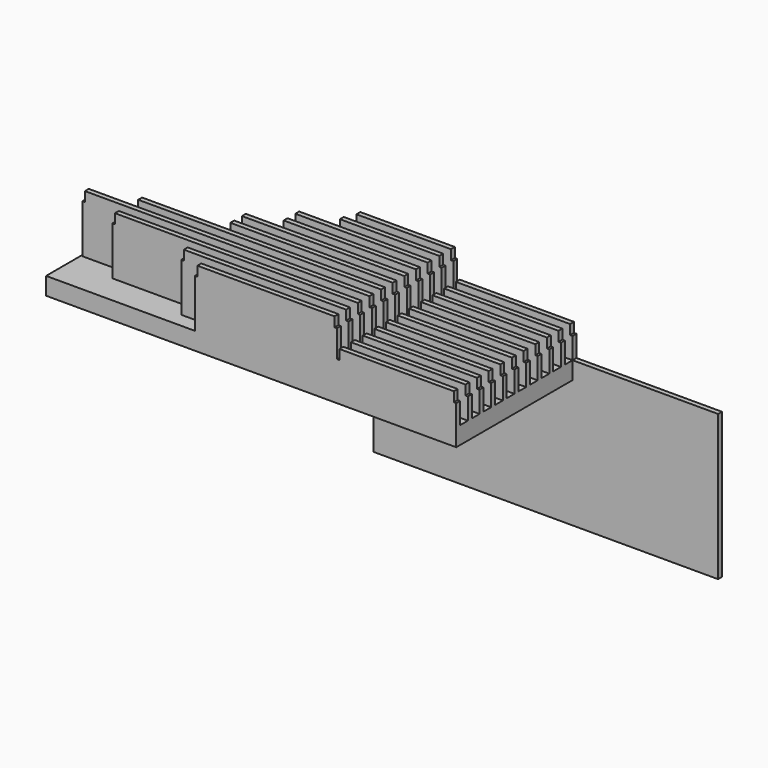
from build123d import *

# Parameters (mm, degrees)
F1_DEPTH  = 123
F2_DEPTH  = 300
F3_R      = 0.5
F4_DEPTH  = 1
F5_W      = 123
F5_H      = 28
F6_DEPTH  = 300
F7_W      = 2.5
F7_H      = 10
F8_DEPTH  = 300
F9_W      = 150
F9_H      = 150
F10_DEPTH = 5
F11_W     = 5
F11_H     = 60
F12_DEPTH = 197.5
F13_W     = 20
F13_H     = 60
F14_DEPTH = 158.5
F15_W     = 20
F15_H     = 60
F15_W_2   = 5
F16_DEPTH = 127.5
F17_W     = 5
F17_H     = 60
F18_DEPTH = 44.5
F19_W     = 5
F19_H     = 60
F20_DEPTH = 1.5
F21_W     = 5
F21_H     = 60
F22_DEPTH = 153.5
F23_W     = 5
F23_H     = 10
F24_DEPTH = 2.5
F25_W     = 5
F25_H     = 10
F26_DEPTH = 2.5
F27_W     = 5
F27_H     = 10
F28_DEPTH = 2.5
F29_W     = 5
F29_H     = 10
F30_DEPTH = 2.5
F31_W     = 5
F31_H     = 10
F32_DEPTH = 2.5
F33_W     = 5
F33_H     = 10
F34_DEPTH = 2.5
F35_W     = 5
F35_H     = 10
F36_DEPTH = 2.5
F37_W     = 5
F37_H     = 10
F38_DEPTH = 2.5
F39_W     = 5
F39_H     = 10
F40_DEPTH = 2.5
F41_W     = 5
F41_H     = 10
F42_DEPTH = 2.5
F43_W     = 5
F43_H     = 10
F44_DEPTH = 2.5
F45_W     = 217.5729006529
F45_H     = 131.9425046444
F46_DEPTH = 5


# Not quite as in the source:
# - a feature names something its author has since deleted; it is built from what else it names


with BuildPart() as f1:
    # F0 (on Right) → F1 (new body)
    with BuildSketch(Plane.YZ):
        Polygon((179.2768240368, 60), (174.2768240368, 60), (174.2768240368, -18.0574953556), (324.2768240368, -18.0574953556), (324.2768240368, -150), (329.2768240368, -150), (329.2768240368, 60), (324.2768240368, 60), (324.2768240368, 0), (314.2768240368, 0), (314.2768240368, 60), (309.2768240368, 60), (309.2768240368, 0), (299.2768240368, 0), (299.2768240368, 60), (294.2768240368, 60), (294.2768240368, 0), (284.2768240368, 0), (284.2768240368, 60), (279.2768240368, 60), (279.2768240368, 0), (269.2768240368, 0), (269.2768240368, 60), (264.2768240368, 60), (264.2768240368, 0), (254.2768240368, 0), (254.2768240368, 60), (249.2768240368, 60), (249.2768240368, 0), (239.2768240368, 0), (239.2768240368, 60), (234.2768240368, 60), (234.2768240368, 0), (224.2768240368, 0), (224.2768240368, 60), (219.2768240368, 60), (219.2768240368, 0), (209.2768240368, 0), (209.2768240368, 60), (204.2768240368, 60), (204.2768240368, 0), (194.2768240368, 0), (194.2768240368, 60), (189.2768240368, 60), (189.2768240368, 0), (179.2768240368, 0), align=None)
    extrude(amount=F1_DEPTH)

    # F0 (on Right) → F2 (join)
    with BuildSketch(Plane.YZ):
        Polygon((179.2768240368, 60), (174.2768240368, 60), (174.2768240368, -18.0574953556), (324.2768240368, -18.0574953556), (324.2768240368, -150), (329.2768240368, -150), (329.2768240368, 60), (324.2768240368, 60), (324.2768240368, 0), (314.2768240368, 0), (314.2768240368, 60), (309.2768240368, 60), (309.2768240368, 0), (299.2768240368, 0), (299.2768240368, 60), (294.2768240368, 60), (294.2768240368, 0), (284.2768240368, 0), (284.2768240368, 60), (279.2768240368, 60), (279.2768240368, 0), (269.2768240368, 0), (269.2768240368, 60), (264.2768240368, 60), (264.2768240368, 0), (254.2768240368, 0), (254.2768240368, 60), (249.2768240368, 60), (249.2768240368, 0), (239.2768240368, 0), (239.2768240368, 60), (234.2768240368, 60), (234.2768240368, 0), (224.2768240368, 0), (224.2768240368, 60), (219.2768240368, 60), (219.2768240368, 0), (209.2768240368, 0), (209.2768240368, 60), (204.2768240368, 60), (204.2768240368, 0), (194.2768240368, 0), (194.2768240368, 60), (189.2768240368, 60), (189.2768240368, 0), (179.2768240368, 0), align=None)
    extrude(amount=-F2_DEPTH)

    # F3 (on face) → F4, piece 2 (join)
    with BuildSketch(Plane(origin=(0, 329.2768240368, 0), x_dir=(-1, 0, 0), z_dir=(0, 1, 0))):
        with Locations((-83.0557048321, -30)):
            Circle(F3_R)
        with Locations((11.1870197579, -30)):
            Circle(F3_R)
    extrude(amount=F4_DEPTH)

    # F5 (on face) → F6 (cut)
    with BuildSketch(Plane(origin=(0, 329.2768240368, 0), x_dir=(-1, 0, 0), z_dir=(0, 1, 0))):
        with Locations((-61.5, 46)):
            Rectangle(F5_W, F5_H)
    extrude(amount=-F6_DEPTH, mode=Mode.SUBTRACT)

    # F7 (on face) → F8 (cut)
    with BuildSketch(Plane(origin=(0, 329.2768240368, 0), x_dir=(-1, 0, 0), z_dir=(0, 1, 0))):
        with Locations((-1.25, 27)):
            Rectangle(F7_W, F7_H)
        with Locations((1.25, 55)):
            Rectangle(F7_W, F7_H)
        with Locations((-121.75, 27)):
            Rectangle(F7_W, F7_H)
    extrude(amount=-F8_DEPTH, mode=Mode.SUBTRACT)



with BuildPart() as f4:
    # F3 (on face) → F4 (new body)
    with BuildSketch(Plane(origin=(0, 329.2768240368, 0), x_dir=(-1, 0, 0), z_dir=(0, 1, 0))):
        with Locations((-203.3374607563, -30)):
            Circle(F3_R)
    extrude(amount=F4_DEPTH)


with BuildPart() as f1_1:
    add(f1.part)

    add(f4.part)  # F10 merges F4
    # F9 (on face) → F10 (join)
    with BuildSketch(Plane(origin=(0, 329.2768240368, 0), x_dir=(-1, 0, 0), z_dir=(0, 1, 0))):
        with Locations((-198, -75)):
            Rectangle(F9_W, F9_H)
    extrude(amount=-F10_DEPTH)

    # F11 (on face) → F12 (cut)
    with BuildSketch(Plane(origin=(-300, 0, 0), x_dir=(0, -1, 0), z_dir=(-1, 0, 0))):
        with Locations((-326.7768240368, 30)):
            Rectangle(F11_W, F11_H)
        with Locations((-311.7768240368, 30)):
            Rectangle(F11_W, F11_H)
    extrude(amount=-F12_DEPTH, mode=Mode.SUBTRACT)

    # F13 (on face) → F14 (cut)
    with BuildSketch(Plane(origin=(-300, 0, 0), x_dir=(0, -1, 0), z_dir=(-1, 0, 0))):
        with Locations((-289.2768240368, 30)):
            Rectangle(F13_W, F13_H)
    extrude(amount=-F14_DEPTH, mode=Mode.SUBTRACT)

    # F15 (on face) → F16 (cut)
    with BuildSketch(Plane(origin=(-300, 0, 0), x_dir=(0, -1, 0), z_dir=(-1, 0, 0))):
        with Locations((-259.2768240368, 30)):
            Rectangle(F15_W, F15_H)
        with Locations((-191.7768240368, 30)):
            Rectangle(F15_W_2, F15_H)
    extrude(amount=-F16_DEPTH, mode=Mode.SUBTRACT)

    # F17 (on face) → F18 (cut)
    with BuildSketch(Plane(origin=(-300, 0, 0), x_dir=(0, -1, 0), z_dir=(-1, 0, 0))):
        with Locations((-236.7768240368, 30)):
            Rectangle(F17_W, F17_H)
        with Locations((-206.7768240368, 30)):
            Rectangle(F17_W, F17_H)
    extrude(amount=-F18_DEPTH, mode=Mode.SUBTRACT)

    # F19 (on face) → F20 (cut)
    with BuildSketch(Plane(origin=(-300, 0, 0), x_dir=(0, -1, 0), z_dir=(-1, 0, 0))):
        with Locations((-221.7768240368, 30)):
            Rectangle(F19_W, F19_H)
    extrude(amount=-F20_DEPTH, mode=Mode.SUBTRACT)

    # F21 (on face) → F22 (cut)
    with BuildSketch(Plane(origin=(-300, 0, 0), x_dir=(0, -1, 0), z_dir=(-1, 0, 0))):
        with Locations((-176.7768240368, 30)):
            Rectangle(F21_W, F21_H)
    extrude(amount=-F22_DEPTH, mode=Mode.SUBTRACT)

    # F23 (on face) → F24 (cut)
    with BuildSketch(Plane(origin=(-298.5, 0, 0), x_dir=(0, -1, 0), z_dir=(-1, 0, 0))):
        with Locations((-221.7768240368, 55)):
            Rectangle(F23_W, F23_H)
    extrude(amount=-F24_DEPTH, mode=Mode.SUBTRACT)

    # F25 (on face) → F26 (cut)
    with BuildSketch(Plane(origin=(-255.5, 0, 0), x_dir=(0, -1, 0), z_dir=(-1, 0, 0))):
        with Locations((-236.7768240368, 55)):
            Rectangle(F25_W, F25_H)
    extrude(amount=-F26_DEPTH, mode=Mode.SUBTRACT)

    # F27 (on face) → F28 (cut)
    with BuildSketch(Plane(origin=(-255.5, 0, 0), x_dir=(0, -1, 0), z_dir=(-1, 0, 0))):
        with Locations((-206.7768240368, 55)):
            Rectangle(F27_W, F27_H)
    extrude(amount=-F28_DEPTH, mode=Mode.SUBTRACT)

    # F29 (on face) → F30 (cut)
    with BuildSketch(Plane(origin=(-172.5, 0, 0), x_dir=(0, -1, 0), z_dir=(-1, 0, 0))):
        with Locations((-251.7768240368, 55)):
            Rectangle(F29_W, F29_H)
    extrude(amount=-F30_DEPTH, mode=Mode.SUBTRACT)

    # F31 (on face) → F32 (cut)
    with BuildSketch(Plane(origin=(-172.5, 0, 0), x_dir=(0, -1, 0), z_dir=(-1, 0, 0))):
        with Locations((-191.7768240368, 55)):
            Rectangle(F31_W, F31_H)
    extrude(amount=-F32_DEPTH, mode=Mode.SUBTRACT)

    # F33 (on face) → F34 (cut)
    with BuildSketch(Plane(origin=(-172.5, 0, 0), x_dir=(0, -1, 0), z_dir=(-1, 0, 0))):
        with Locations((-266.7768240368, 55)):
            Rectangle(F33_W, F33_H)
    extrude(amount=-F34_DEPTH, mode=Mode.SUBTRACT)

    # F35 (on face) → F36 (cut)
    with BuildSketch(Plane(origin=(-146.5, 0, 0), x_dir=(0, -1, 0), z_dir=(-1, 0, 0))):
        with Locations((-176.7768240368, 55)):
            Rectangle(F35_W, F35_H)
    extrude(amount=-F36_DEPTH, mode=Mode.SUBTRACT)

    # F37 (on face) → F38 (cut)
    with BuildSketch(Plane(origin=(-141.5, 0, 0), x_dir=(0, -1, 0), z_dir=(-1, 0, 0))):
        with Locations((-281.7768240368, 55)):
            Rectangle(F37_W, F37_H)
    extrude(amount=-F38_DEPTH, mode=Mode.SUBTRACT)

    # F39 (on face) → F40 (cut)
    with BuildSketch(Plane(origin=(-141.5, 0, 0), x_dir=(0, -1, 0), z_dir=(-1, 0, 0))):
        with Locations((-296.7768240368, 55)):
            Rectangle(F39_W, F39_H)
    extrude(amount=-F40_DEPTH, mode=Mode.SUBTRACT)

    # F41 (on face) → F42 (join)
    with BuildSketch(Plane(origin=(-102.5, 0, 0), x_dir=(0, -1, 0), z_dir=(-1, 0, 0))):
        with Locations((-311.7768240368, 55)):
            Rectangle(F41_W, F41_H)
    extrude(amount=F42_DEPTH)

    # F43 (on face) → F44 (cut)
    with BuildSketch(Plane(origin=(-102.5, 0, 0), x_dir=(0, -1, 0), z_dir=(-1, 0, 0))):
        with Locations((-326.7768240368, 55)):
            Rectangle(F43_W, F43_H)
    extrude(amount=-F44_DEPTH, mode=Mode.SUBTRACT)

    # F45 (on face) → F46 (cut)
    with BuildSketch(Plane(origin=(0, 329.2768240368, 0), x_dir=(-1, 0, 0), z_dir=(0, 1, 0))):
        with Locations((191.2135496736, -84.0287476778)):
            Rectangle(F45_W, F45_H)
    extrude(amount=-F46_DEPTH, mode=Mode.SUBTRACT)


solid = f1_1.part
